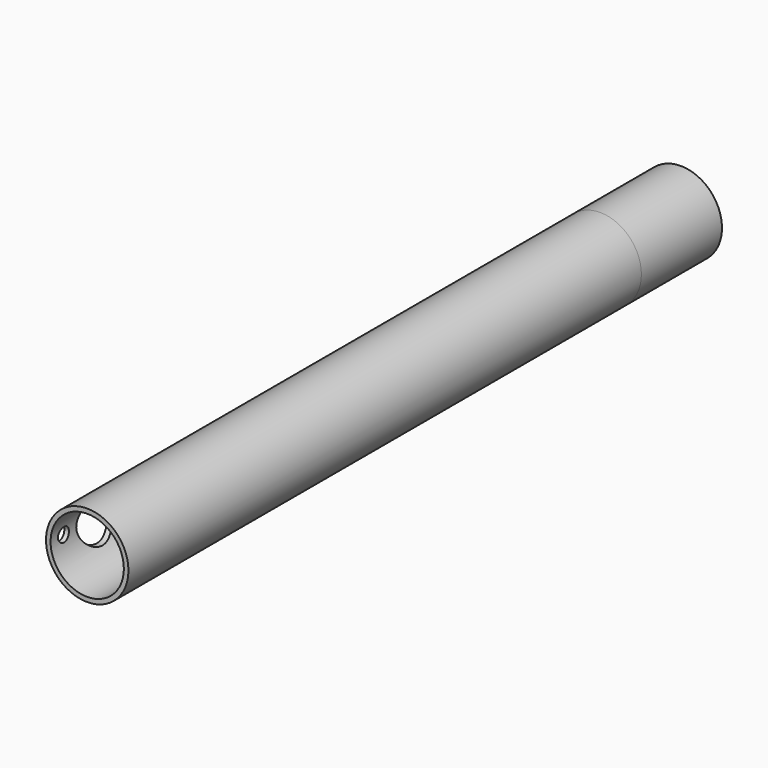
from build123d import *

# Parameters (mm, degrees)
F3_R      = 4.5
F4_DEPTH  = 60.5
F8_DEPTH  = 60.5
F6_R      = 4.5
F6_R_2    = 4
F9_DEPTH  = 9.5
F7_R      = 4.5
F7_R_2    = 4
F10_DEPTH = 11
F11_R     = 2.5
F11_R_2   = 0.75
F12_DEPTH = 4.501


# Not quite as in the source:
# - ends of sketch curves that miss each other by under 0.0002 mm in the source are joined


with BuildPart() as f4:
    # F3 (on Front) → F4 (new body)
    with BuildSketch(Plane.XZ):
        Circle(F3_R)
    extrude(amount=F4_DEPTH)

    # F5 (on face) → F8 (cut, through all)
    with BuildSketch(Plane.XZ.offset(60.5)):
        with BuildLine():
            Line((-1.25, -3.8), (0, -3.8))
            Line((0, -3.8), (1.25, -3.8))
            Line((1.25, -3.8), (1.25, -3.7))
            ThreePointArc((1.25, -3.7), (1.3085786438, -3.5585786438), (1.45, -3.5))
            Line((1.45, -3.5), (2, -3.5))
            Line((2, -3.5), (2, -3.05))
            ThreePointArc((2, -3.05), (2.0585786438, -2.9085786438), (2.2, -2.85))
            Line((2.2, -2.85), (3.15, -2.85))
            Line((3.15, -2.85), (3.15, -2.15))
            Line((3.15, -2.15), (2.2, -2.15))
            ThreePointArc((2.2, -2.15), (2.0585786438, -2.0914213562), (2, -1.95))
            Line((2, -1.95), (2, -1.887459))
            ThreePointArc((2, -1.887459), (2.1033535752, -1.771554046), (2.2, -1.65))
            Line((2.2, -1.65), (3.75, -1.65))
            Line((3.75, -1.65), (3.75, 0))
            Line((3.75, 0), (3.75, 1.65))
            Line((3.75, 1.65), (2.2, 1.65))
            ThreePointArc((2.2, 1.65), (2.1033535752, 1.771554046), (1.9999998047, 1.8874588157))
            Line((1.9999998047, 1.8874588157), (2, 1.95))
            ThreePointArc((2, 1.95), (2.0585786438, 2.0914213562), (2.2, 2.15))
            Line((2.2, 2.15), (3.15, 2.15))
            Line((3.15, 2.15), (3.15, 2.85))
            Line((3.15, 2.85), (2.2, 2.85))
            ThreePointArc((2.2, 2.85), (2.0585786438, 2.9085786438), (2, 3.05))
            Line((2, 3.05), (2, 3.5))
            Line((2, 3.5), (1.45, 3.5))
            ThreePointArc((1.45, 3.5), (1.3085786438, 3.5585786438), (1.25, 3.7))
            Line((1.25, 3.7), (1.25, 3.8))
            Line((1.25, 3.8), (0, 3.8))
            Line((0, 3.8), (-1.25, 3.8))
            Line((-1.25, 3.8), (-1.25, 3.7))
            ThreePointArc((-1.25, 3.7), (-1.3085786438, 3.5585786438), (-1.45, 3.5))
            Line((-1.45, 3.5), (-2, 3.5))
            Line((-2, 3.5), (-2, 3.05))
            ThreePointArc((-2, 3.05), (-2.0585786438, 2.9085786438), (-2.2, 2.85))
            Line((-2.2, 2.85), (-3.15, 2.85))
            Line((-3.15, 2.85), (-3.15, 2.15))
            Line((-3.15, 2.15), (-2.2, 2.15))
            ThreePointArc((-2.2, 2.15), (-2.0585786438, 2.0914213562), (-2, 1.95))
            Line((-2, 1.95), (-2, 1.887459))
            ThreePointArc((-2, 1.887459), (-2.1033535752, 1.771554046), (-2.2, 1.65))
            Line((-2.2, 1.65), (-3.75, 1.65))
            Line((-3.75, 1.65), (-3.75, 0))
            Line((-3.75, 0), (-3.75, -1.65))
            Line((-3.75, -1.65), (-2.2, -1.65))
            ThreePointArc((-2.2, -1.65), (-2.1033535752, -1.771554046), (-1.9999998047, -1.8874588157))
            Line((-1.9999998047, -1.8874588157), (-2, -1.95))
            ThreePointArc((-2, -1.95), (-2.0585786438, -2.0914213562), (-2.2, -2.15))
            Line((-2.2, -2.15), (-3.15, -2.15))
            Line((-3.15, -2.15), (-3.15, -2.85))
            Line((-3.15, -2.85), (-2.2, -2.85))
            ThreePointArc((-2.2, -2.85), (-2.0585786438, -2.9085786438), (-2, -3.05))
            Line((-2, -3.05), (-2, -3.5))
            Line((-2, -3.5), (-1.45, -3.5))
            ThreePointArc((-1.45, -3.5), (-1.3085786438, -3.5585786438), (-1.25, -3.7))
            Line((-1.25, -3.7), (-1.25, -3.8))
        make_face()
    extrude(amount=-F8_DEPTH, mode=Mode.SUBTRACT)

    # F6 (on face) → F9 (join)
    with BuildSketch(Plane.XZ.offset(60.5)):
        Circle(F6_R)
        Circle(F6_R_2, mode=Mode.SUBTRACT)
    extrude(amount=F9_DEPTH)

    # F7 (on face) → F10 (join)
    with BuildSketch(Plane(origin=(0, 0, 0), x_dir=(-1, 0, 0), z_dir=(0, 1, 0))):
        Circle(F7_R)
        Circle(F7_R_2, mode=Mode.SUBTRACT)
    extrude(amount=F10_DEPTH)

    # F11 (on Right) → F12 (cut, through all)
    with BuildSketch(Plane.YZ):
        with Locations((-64, 0)):
            Circle(F11_R)
        with Locations((-68.25, 0)):
            Circle(F11_R_2)
    extrude(amount=-F12_DEPTH, mode=Mode.SUBTRACT)


solid = f4.part
